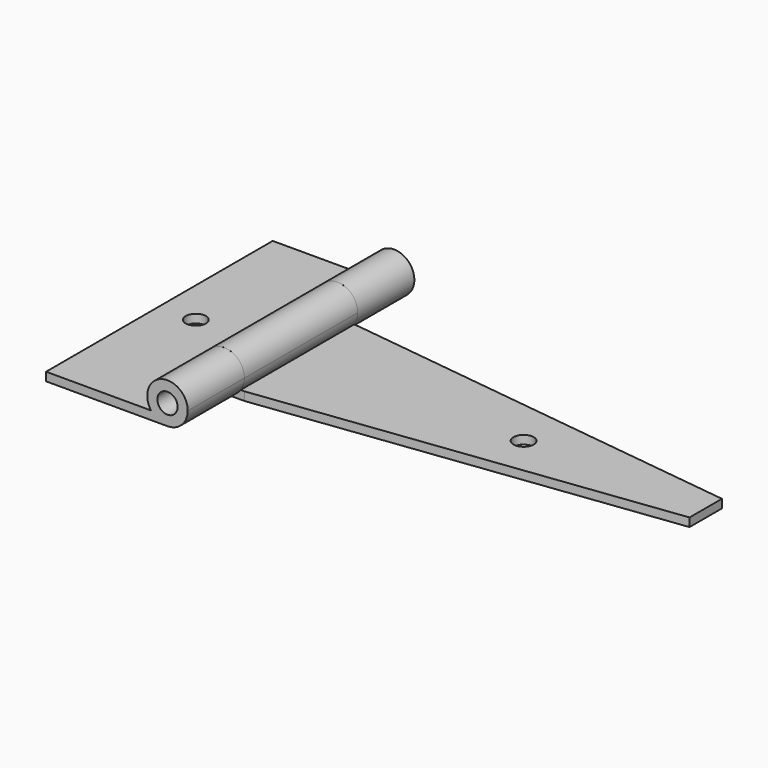
from build123d import *

# Parameters (mm, degrees)
F1_DEPTH  = 2.667
F2_DEPTH  = 6.35
F4_DEPTH  = 44.45
F5_R      = 3.175
F6_DEPTH  = 44.45
F8_DEPTH  = 2.667
F9_W      = 22.225
F9_H      = 2.667
F10_DEPTH = 6.35
F11_R     = 3.175
F12_DEPTH = 22.225
F13_R     = 3.175
F14_DEPTH = 22.225
F15_R     = 3.175
F16_DEPTH = 25.4
F17_R     = 3.175
F18_DEPTH = 25.4


with BuildPart() as f1:
    # F0 (on Top) → F1 (new body)
    with BuildSketch(Plane.XY):
        Polygon((127, 6.35), (0, 22.225), (0, -22.225), (127, -6.35), align=None)
    extrude(amount=F1_DEPTH)

    # F2 (add): a face of the model
    f2_faces = [f1.faces().sort_by_distance(p)[0] for p in [
        (0, 0, 1.3335),
    ]]
    extrude(f2_faces, amount=F2_DEPTH)

    # F3 (on face) → F4 (join, through all)
    with BuildSketch(Plane.XZ.offset(22.225)):
        with BuildLine():
            ThreePointArc((-1.177185389, 2.667), (-0.3014517122, 4.4167220557), (0, 6.35))
            ThreePointArc((0, 6.35), (-10.8401280605, 10.8401280605), (-6.35, 0))
            Line((-6.35, 0), (-6.35, 2.667))
            Line((-6.35, 2.667), (-1.177185389, 2.667))
        make_face()
    extrude(amount=-F4_DEPTH)

    # F5 (on face) → F6 (cut, through all)
    with BuildSketch(Plane.XZ.offset(22.225)):
        with Locations((-6.35, 6.35)):
            Circle(F5_R)
    extrude(amount=-F6_DEPTH, mode=Mode.SUBTRACT)

    # F17 (on face) → F18 (cut)
    with BuildSketch(Plane.XY.offset(2.667)):
        with Locations((69.85, 0)):
            Circle(F17_R)
    extrude(amount=-F18_DEPTH, mode=Mode.SUBTRACT)


with BuildPart() as f8:
    # F7 (on Top) → F8 (new body)
    with BuildSketch(Plane.XY):
        Polygon((-12.7, -44.45), (-12.7, -38.1), (-12.7, 38.1), (-12.7, 44.45), (-44.45, 44.45), (-44.45, -44.45), align=None)
    extrude(amount=F8_DEPTH)

    # F9 (on face) → F10 (join)
    with BuildSketch(Plane.YZ.offset(-12.7)):
        with Locations((-33.3375, 1.3335)):
            Rectangle(F9_W, F9_H)
        with Locations((33.3375, 1.3335)):
            Rectangle(F9_W, F9_H)
    extrude(amount=F10_DEPTH)

    # F11 (on face) → F12 (join, through all)
    with BuildSketch(Plane.XZ.offset(44.45)):
        with BuildLine():
            Line((-6.35, 2.667), (-6.35, 0))
            ThreePointArc((-6.35, 0), (-1.8598719395, 1.8598719395), (0, 6.35))
            ThreePointArc((0, 6.35), (-8.2832779443, 12.3985482878), (-11.522814611, 2.667))
            Line((-11.522814611, 2.667), (-6.35, 2.667))
        make_face()
        with Locations((-6.35, 6.35)):
            Circle(F11_R, mode=Mode.SUBTRACT)
    extrude(amount=-F12_DEPTH)

    # F13 (on face) → F14 (join, through all)
    with BuildSketch(Plane(origin=(0, 44.45, 0), x_dir=(-1, 0, 0), z_dir=(0, 1, 0))):
        with BuildLine():
            ThreePointArc((11.522814611, 2.667), (12.3985482878, 4.4167220557), (12.7, 6.35))
            ThreePointArc((12.7, 6.35), (1.8598719395, 10.8401280605), (6.35, 0))
            Line((6.35, 0), (6.35, 2.667))
            Line((6.35, 2.667), (11.522814611, 2.667))
        make_face()
        with Locations((6.35, 6.35)):
            Circle(F13_R, mode=Mode.SUBTRACT)
    extrude(amount=-F14_DEPTH)

    # F15 (on face) → F16 (cut)
    with BuildSketch(Plane.XY.offset(2.667)):
        with Locations((-33.02, 0)):
            Circle(F15_R)
    extrude(amount=-F16_DEPTH, mode=Mode.SUBTRACT)


solid = Compound([f1.part, f8.part])
